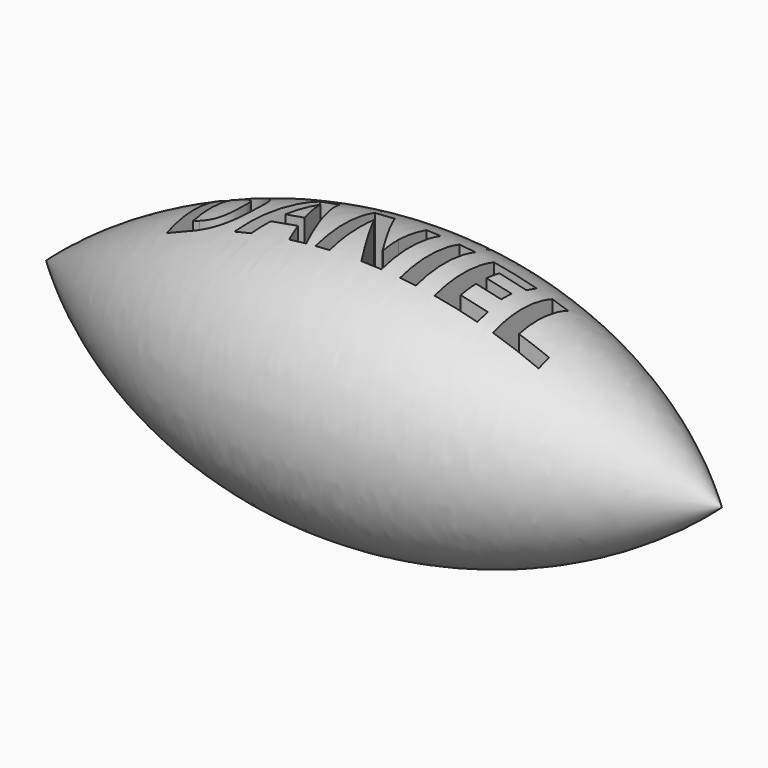
from build123d import *

# Parameters (mm, degrees)
F2_TEXT_SIZE = 23.3615050092
F3_DEPTH     = 29.0681467697


# Not quite as in the source:
# - Text() gives the source's letters only with a copy of the font that has no kerning and outlines rounded to 1/6400 em; it was checked with that copy


with BuildPart() as f1:
    # F0 (on Top) → F1 (revolve)
    with BuildSketch(Plane.XY):
        with BuildLine():
            Line((76.4868333936, 0), (-74.5307491157, -0.8492235475))
            ThreePointArc((-74.5307491157, -0.8492235475), (1.1414940677, -29.491298874), (76.4868333936, 0))
        make_face()
    revolve(axis=Axis((0.9780421389, -0.4246117737, 0), (0.9999841894, 0.0056232533, 0)))

    # F2 (on Top) → F3 (cut, through all)
    with BuildSketch(Plane.XY):
        with Locations((-43.5281693935, -8.4101418033)):
            Text('DANIEL', F2_TEXT_SIZE, font='Open Sans', font_style=FontStyle.BOLD, text_align=(TextAlign.LEFT, TextAlign.BOTTOM))
    extrude(amount=F3_DEPTH, mode=Mode.SUBTRACT)


solid = f1.part
